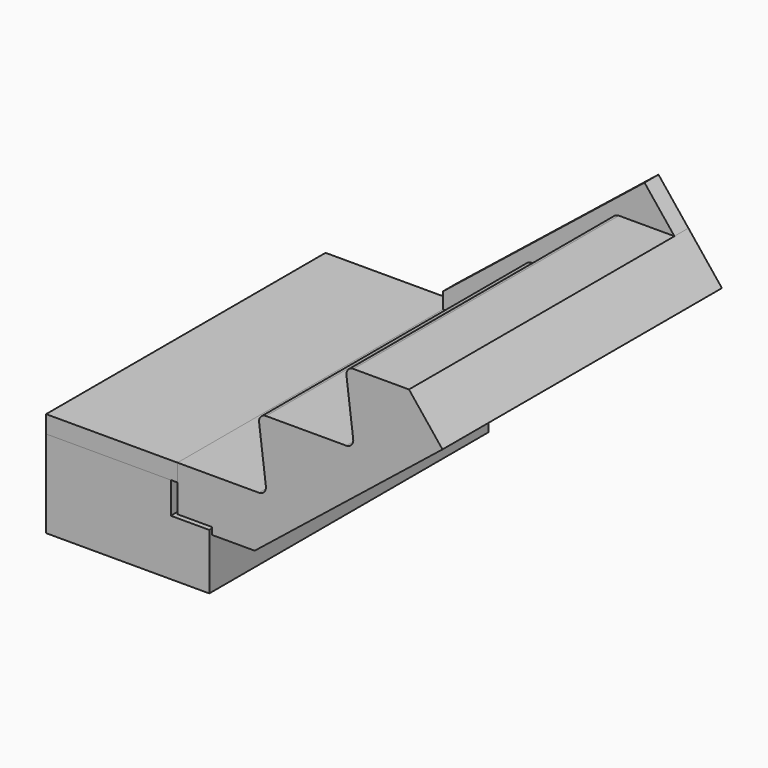
from build123d import *

# Parameters (mm, degrees)
F1_DEPTH = 1000
F2_DEPTH = 50
F3_DEPTH = 1000
F4_DEPTH = 1000


# Not quite as in the source:
# - ends of sketch curves that miss each other by under 0.0002 mm in the source are joined


with BuildPart() as f1:
    # F0 (on Front) → F1 (new body)
    with BuildSketch(Plane.XZ):
        with BuildLine():
            Line((-21.236031, -90.492915), (-254.343951, -90.492915))
            Line((-254.343951, -90.492915), (-254.343951, -140.492915))
            Line((-254.343951, -140.492915), (-254.343951, -220.492915))
            Line((-254.343951, -220.492915), (-155.429775, -220.492915))
            Line((-155.429775, -220.492915), (-155.429775, -240.492915))
            Line((-155.429775, -240.492915), (-33.408643, -240.492915))
            Line((-33.408643, -240.492915), (154.0913568979, -90.4929148724))
            Line((154.0913568979, -90.4929148724), (504.14619, 189.550952))
            Line((504.14619, 189.550952), (408.249622949, 309.5070849592))
            Line((408.249622949, 309.5070849592), (249.075257, 309.507085))
            ThreePointArc((249.075257, 309.507085), (234.0816933606, 302.7431361252), (229.2296995119, 287.026389939))
            Line((229.2296995119, 287.026389939), (248.609526, 131.987779))
            ThreePointArc((248.609526, 131.987779), (243.7575323111, 116.2710335028), (228.763969, 109.507085))
            Line((228.763969, 109.507085), (-0.924743, 109.507085))
            ThreePointArc((-0.924743, 109.507085), (-15.9183066394, 102.7431361252), (-20.7703004881, 87.026389939))
            Line((-20.7703004881, 87.026389939), (-1.390474, -68.012221))
            ThreePointArc((-1.390474, -68.012221), (-6.2424676889, -83.7289664972), (-21.236031, -90.492915))
        make_face()
    extrude(amount=F1_DEPTH)


with BuildPart() as f2:
    # F0 (on Front) → F2 (new body)
    with BuildSketch(Plane.XZ):
        with BuildLine():
            Line((-254.343951, -44.837372), (-254.343951, -90.492915))
            Line((-254.343951, -90.492915), (-21.236031, -90.492915))
            ThreePointArc((-21.236031, -90.492915), (-6.2424676889, -83.7289664972), (-1.3904733888, -68.0122209236))
            Line((-1.3904733888, -68.0122209236), (-20.7703, 87.02639))
            ThreePointArc((-20.7703, 87.02639), (-15.9183066394, 102.7431361252), (-0.924743, 109.507085))
            Line((-0.924743, 109.507085), (228.763969, 109.507085))
            ThreePointArc((228.763969, 109.507085), (243.7575323111, 116.2710335028), (248.6095266112, 131.9877790764))
            Line((248.6095266112, 131.9877790764), (229.2297, 287.02639))
            ThreePointArc((229.2297, 287.02639), (234.0816933606, 302.7431361252), (249.075257, 309.507085))
            Line((249.075257, 309.507085), (408.249623, 309.507085))
            Line((408.249623, 309.507085), (322.5647089299, 416.689554944))
            Line((322.5647089299, 416.689554944), (-254.343951, -44.837372))
        make_face()
    extrude(amount=F2_DEPTH)


with BuildPart() as f3:
    # F0 (on Front) → F3 (new body)
    with BuildSketch(Plane.XZ):
        Polygon((-273.580387, -140.492915), (-630.630191, -140.492915), (-630.630191, -390.492915), (-163.408643, -390.492915), (-163.408643, -230.492915), (-273.580387, -230.492915), align=None)
    extrude(amount=F3_DEPTH)


with BuildPart() as f4:
    # F0 (on Front) → F4 (new body)
    with BuildSketch(Plane.XZ):
        Polygon((-254.343951, -140.492915), (-254.343951, -90.492915), (-630.630191, -90.492915), (-630.630191, -140.492915), (-273.580387, -140.492915), align=None)
    extrude(amount=F4_DEPTH)


solid = Compound([f1.part, f2.part, f3.part, f4.part])
